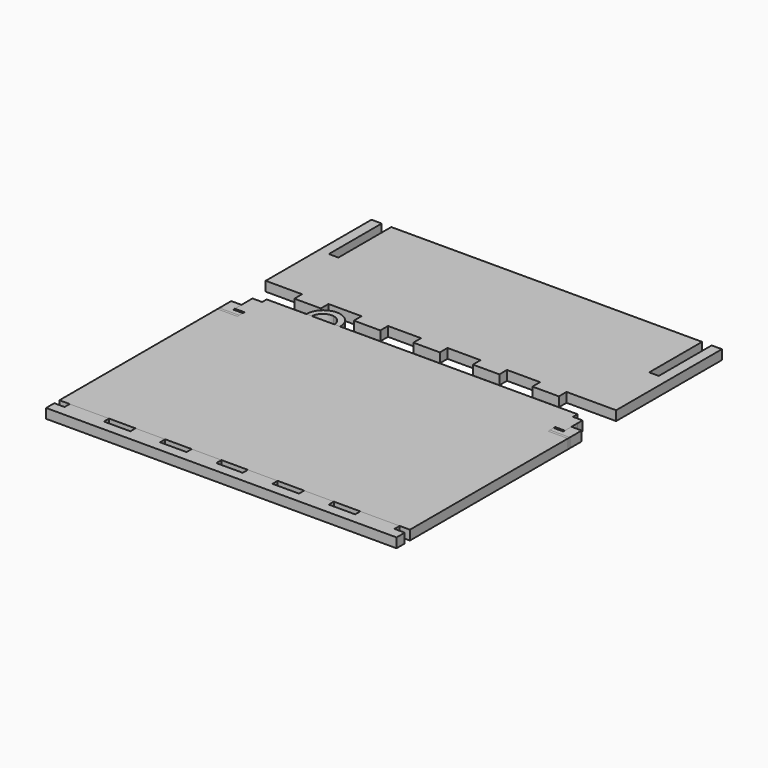
from build123d import *

# Parameters (mm, degrees)
F2_DEPTH  = 2.9
F3_W      = 94
F3_H      = 16
F3_H_2    = 4
F3_W_2    = 3.1
F3_H_3    = 20
F4_DEPTH  = 2.9
F6_DEPTH  = 2.9
F8_DEPTH  = 2.9
F9_W      = 94
F9_H      = 1
F10_DEPTH = 2.9


# Not quite as in the source:
# - ends of sketch curves that miss each other by under 0.0002 mm in the source are joined


with BuildPart() as f2:
    # F1 (on Top) → F2 (new body)
    with BuildSketch(Plane.XY):
        Polygon((-53, -31.9), (-53, -35), (53, -35), (53, -31.9), (49.9, -31.9), (49.9, -29), (53, -29), (53, 35), (49.9, 35), (49.9, 31.9), (47, 31.9), (47, 35), (-47, 35), (-47, 31.9), (-49.9, 31.9), (-49.9, 35), (-53, 35), (-53, -29), (-49.9, -29), (-49.9, -31.9), align=None)
        Polygon((38, 29), (47, 29), (47, 22), (49.9, 22), (49.9, 14), (47, 14), (47, 4), (49.9, 4), (49.9, -4), (47, -4), (47, -14), (49.9, -14), (49.9, -22), (47, -22), (47, -29), (38, -29), (38, -31.9), (30, -31.9), (30, -29), (21, -29), (21, -31.9), (13, -31.9), (13, -29), (4, -29), (4, -31.9), (-4, -31.9), (-4, -29), (-13, -29), (-13, -31.9), (-21, -31.9), (-21, -29), (-30, -29), (-30, -31.9), (-38, -31.9), (-38, -29), (-47, -29), (-47, -22), (-49.9, -22), (-49.9, -14), (-47, -14), (-47, -4), (-49.9, -4), (-49.9, 4), (-47, 4), (-47, 14), (-49.9, 14), (-49.9, 22), (-47, 22), (-47, 29), (-42, 29), (-42, 31.9), (-34, 31.9), (-34, 29), (-24, 29), (-24, 31.9), (-16, 31.9), (-16, 29), (-6, 29), (-6, 31.9), (2, 31.9), (2, 29), (12, 29), (12, 31.9), (20, 31.9), (20, 29), (30, 29), (30, 31.9), (38, 31.9), align=None, mode=Mode.SUBTRACT)
        Polygon((47, -29), (0, 0), (-47, -29), (-38, -29), (-30, -29), (-21, -29), (-13, -29), (-4, -29), (4, -29), (13, -29), (21, -29), (30, -29), (38, -29), align=None)
        Polygon((-47, -29), (0, 0), (-47, 29), (-47, 22), (-47, 14), (-47, 4), (-47, -4), (-47, -14), (-47, -22), align=None)
        Polygon((0, 0), (47, 29), (38, 29), (30, 29), (20, 29), (12, 29), (2, 29), (-6, 29), (-16, 29), (-24, 29), (-34, 29), (-42, 29), (-47, 29), align=None)
        Polygon((47, 22), (47, 29), (0, 0), (47, -29), (47, -22), (47, -14), (47, -4), (47, 4), (47, 14), align=None)
    extrude(amount=F2_DEPTH)


with BuildPart() as f4:
    # F3 (on Top) → F4 (new body)
    with BuildSketch(Plane.XY):
        with Locations((-0.1350676175, 76.1836106628)):
            Rectangle(F3_W, F3_H)
        with Locations((-0.1350676175, 86.1836106628)):
            Rectangle(F3_W, F3_H_2)
        with Locations((-51.5850676175, 78.1836106628)):
            Rectangle(F3_W_2, F3_H_3)
        Polygon((37.8649323825, 48.1836106628), (52.8649323825, 48.1836106628), (52.8649323825, 68.1836106628), (49.7649323825, 68.1836106628), (46.8649323825, 68.1836106628), (-47.1350676175, 68.1836106628), (-50.0350676175, 68.1836106628), (-53.1350676175, 68.1836106628), (-53.1350676175, 48.1836106628), (-42.1350676175, 48.1836106628), (-42.1350676175, 45.2836106628), (-34.1350676175, 45.2836106628), (-34.1350676175, 48.1836106628), (-24.1350676175, 48.1836106628), (-24.1350676175, 45.2836106628), (-16.1350676175, 45.2836106628), (-16.1350676175, 48.1836106628), (-6.1350676175, 48.1836106628), (-6.1350676175, 45.2836106628), (1.8649323825, 45.2836106628), (1.8649323825, 48.1836106628), (11.8649323825, 48.1836106628), (11.8649323825, 45.2836106628), (19.8649323825, 45.2836106628), (19.8649323825, 48.1836106628), (29.8649323825, 48.1836106628), (29.8649323825, 45.2836106628), (37.8649323825, 45.2836106628), align=None)
        with Locations((51.3149323825, 78.1836106628)):
            Rectangle(F3_W_2, F3_H_3)
    extrude(amount=F4_DEPTH)


with BuildPart() as f6:
    # F5 (on Top) → F6 (new body)
    with BuildSketch(Plane.XY):
        Polygon((-29, 20), (-29, 15), (29, 15), (29, 30.9375), (-25.0000005956, 39.3750000931), (-26.689130988, 39.6389267169), (-29, 40), (-30, 40.15625), (-33.3108692899, 40.6735733265), (-35, 40.9375), (-35, -2.9), (-31.9, -2.9), (-31.9, 20), align=None)
        Polygon((-29, 0), (-22, 0), (-22, -2.9), (-14, -2.9), (-14, 0), (-4, 0), (-4, -2.9), (4, -2.9), (4, 0), (14, 0), (14, -2.9), (22, -2.9), (22, 0), (35, 0), (35, 15), (31.9, 15), (29, 15), (-29, 15), align=None)
        Polygon((31.9, 30.484375), (31.9, 15), (35, 15), (35, 30), align=None)
        with BuildLine():
            Line((-26.689130988, 39.6389267169), (-25.0000005956, 39.3750000931))
            ThreePointArc((-25.0000005956, 39.3750000931), (-29.0872008599, 45.9981668051), (-35, 40.9375))
            Line((-35, 40.9375), (-33.3108692899, 40.6735733265))
            ThreePointArc((-33.3108692899, 40.6735733265), (-32.1483227603, 43.3077928719), (-29.3824919046, 44.1082986104))
            ThreePointArc((-29.3824919046, 44.1082986104), (-26.9926904447, 42.5022249342), (-26.689130988, 39.6389267169))
        make_face()
    extrude(amount=F6_DEPTH)


with BuildPart() as f8:
    # F7 (on Top) → F8 (new body)
    with BuildSketch(Plane.XY):
        with BuildLine():
            Line((-47, 0), (-38, 0))
            Line((-38, 0), (-38, -2.9))
            Line((-38, -2.9), (-30, -2.9))
            Line((-30, -2.9), (-30, 0))
            Line((-30, 0), (-21, 0))
            Line((-21, 0), (-21, -2.9))
            Line((-21, -2.9), (-13, -2.9))
            Line((-13, -2.9), (-13, 0))
            Line((-13, 0), (-4, 0))
            Line((-4, 0), (-4, -2.9))
            Line((-4, -2.9), (4, -2.9))
            Line((4, -2.9), (4, 0))
            Line((4, 0), (13, 0))
            Line((13, 0), (13, -2.9))
            Line((13, -2.9), (21, -2.9))
            Line((21, -2.9), (21, 0))
            Line((21, 0), (30, 0))
            Line((30, 0), (30, -2.9))
            Line((30, -2.9), (38, -2.9))
            Line((38, -2.9), (38, 0))
            Line((38, 0), (47, 0))
            Line((47, 0), (47, 15))
            Line((47, 15), (49.9, 15))
            Line((49.9, 15), (49.9, -2.9))
            Line((49.9, -2.9), (53, -2.9))
            Line((53, -2.9), (53, 30.5))
            Line((53, 30.5), (9, 30.5))
            Line((9, 30.5), (9, 11))
            ThreePointArc((9, 11), (7.8284271247, 8.1715728753), (5, 7))
            Line((5, 7), (0, 7))
            Line((0, 7), (-5, 7))
            ThreePointArc((-5, 7), (-7.8284271247, 8.1715728753), (-9, 11))
            Line((-9, 11), (-9, 30.5))
            Line((-9, 30.5), (-53, 30.5))
            Line((-53, 30.5), (-53, -2.9))
            Line((-53, -2.9), (-49.9, -2.9))
            Line((-49.9, -2.9), (-49.9, 15))
            Line((-49.9, 15), (-47, 15))
            Line((-47, 15), (-47, 0))
        make_face()
        with BuildLine():
            Line((0, 30.5), (-9, 30.5))
            Line((-9, 30.5), (-9, 11))
            ThreePointArc((-9, 11), (-7.8284271247, 8.1715728753), (-5, 7))
            Line((-5, 7), (0, 7))
            Line((0, 7), (0, 30.5))
        make_face()
        with BuildLine():
            Line((9, 30.5), (0, 30.5))
            Line((0, 30.5), (0, 7))
            Line((0, 7), (5, 7))
            ThreePointArc((5, 7), (7.8284271247, 8.1715728753), (9, 11))
            Line((9, 11), (9, 30.5))
        make_face()
    extrude(amount=F8_DEPTH)


with BuildPart() as f10:
    # F9 (on Top) → F10 (new body)
    with BuildSketch(Plane.XY):
        Polygon((49.917257, 37.184827), (47, 37.190595), (47, 34.48852), (49.911914, 34.482763), align=None)
        Polygon((-47, 37.190595), (-47, 39.190599), (-49.921211, 39.184823), (-49.9172566996, 37.1848270006), align=None)
        Polygon((47, 39.190599), (47, 40.900225), (-47, 40.900225), (-47, 39.190599), (-47, 37.190595), (-47, 34.48852), (-47, 32.488516), (-47, 30.778891), (47, 30.778891), (47, 32.488516), (47, 34.48852), (47, 37.190595), align=None)
        Polygon((53, 29.778891), (47, 29.778891), (-47, 29.778891), (-53, 29.778891), (-53, -29.949115), (53, -29.949115), align=None)
        with Locations((0, 30.278891)):
            Rectangle(F9_W, F9_H)
        Polygon((-47, 34.48852), (-47, 37.190595), (-49.917257, 37.184827), (-49.9119143024, 34.4827629994), align=None)
        Polygon((49.921211, 39.184823), (47, 39.190599), (47, 37.190595), (49.917257, 37.184827), align=None)
        Polygon((-47, 32.488516), (-47, 34.48852), (-49.911914, 34.482763), (-49.90796, 32.482766), align=None)
        Polygon((49.911914, 34.482763), (47, 34.48852), (47, 32.488516), (49.90796, 32.482766), align=None)
    extrude(amount=F10_DEPTH)


solid = Compound([f2.part, f4.part, f6.part, f8.part, f10.part])
